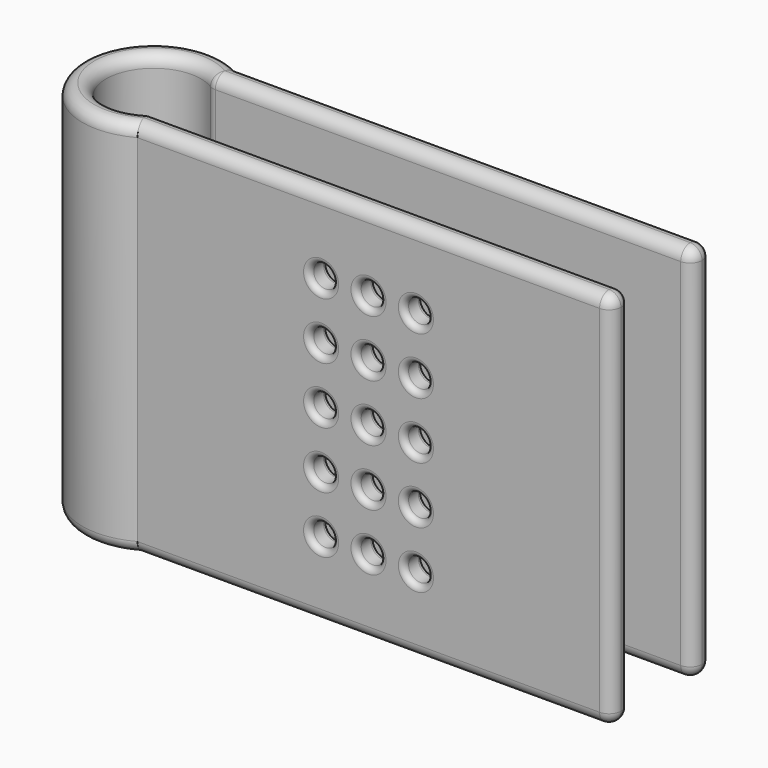
from build123d import *

# Parameters (mm, degrees)
F1_DEPTH = 25.4
F2_R     = 0.79374
F3_R     = 0.79375
F4_DEPTH = 8.9518078406
F5_R     = 0.381


# Not quite as in the source:
# - a fillet or chamfer is up to 0.001 mm smaller than in the source, because OpenCascade refuses the exact size


with BuildPart() as f1:
    # F0 (on Top) → F1 (new body)
    with BuildSketch(Plane.XY):
        with BuildLine():
            ThreePointArc((1.8211051854, -2.6008077406), (-3.175, 0), (1.8211051854, 2.6008077406))
            Line((1.8211051854, 2.6008077406), (2.7316577781, 3.9012116109))
            ThreePointArc((2.7316577781, 3.9012116109), (2.5034693369, 4.0514253701), (2.2670431226, 4.1883077406))
            ThreePointArc((2.2670431226, 4.1883077406), (-4.7625, 0), (2.2670431226, -4.1883077406))
            ThreePointArc((2.2670431226, -4.1883077406), (2.5034693369, -4.0514253701), (2.7316577781, -3.9012116109))
            Line((2.7316577781, -3.9012116109), (1.8211051854, -2.6008077406))
        make_face()
        with BuildLine():
            ThreePointArc((2.2670431226, 4.1883077406), (2.5034693369, 4.0514253701), (2.7316577781, 3.9012116109))
            ThreePointArc((2.7316577781, 3.9012116109), (3.4229686317, 3.3112976303), (3.989637245, 2.6008077406))
            Line((3.989637245, 2.6008077406), (34.0170431226, 2.6008077406))
            Line((34.0170431226, 2.6008077406), (34.0170431226, 4.1883077406))
            Line((34.0170431226, 4.1883077406), (2.2670431226, 4.1883077406))
        make_face()
        with BuildLine():
            Line((3.989637245, -2.6008077406), (1.8211051854, -2.6008077406))
            Line((1.8211051854, -2.6008077406), (2.7316577781, -3.9012116109))
            ThreePointArc((2.7316577781, -3.9012116109), (3.4229686317, -3.3112976303), (3.989637245, -2.6008077406))
        make_face()
        with BuildLine():
            ThreePointArc((3.989637245, -2.6008077406), (3.4229686317, -3.3112976303), (2.7316577781, -3.9012116109))
            ThreePointArc((2.7316577781, -3.9012116109), (2.5034693369, -4.0514253701), (2.2670431226, -4.1883077406))
            Line((2.2670431226, -4.1883077406), (34.0170431226, -4.1883077406))
            Line((34.0170431226, -4.1883077406), (34.0170431226, -2.6008077406))
            Line((34.0170431226, -2.6008077406), (3.989637245, -2.6008077406))
        make_face()
        with BuildLine():
            Line((2.7316577781, 3.9012116109), (1.8211051854, 2.6008077406))
            Line((1.8211051854, 2.6008077406), (3.989637245, 2.6008077406))
            ThreePointArc((3.989637245, 2.6008077406), (3.4229686317, 3.3112976303), (2.7316577781, 3.9012116109))
        make_face()
    extrude(amount=F1_DEPTH)

    # F2 (radius 0.79375 in the source; OpenCascade refuses exactly that, so slightly less here)
    f2_edges = [f1.edges().sort_by_distance(p)[0] for p in [
        (-3.175, 0, 25.4),
        (17.919074, 2.600808, 25.4),
        (34.017043, 3.394558, 25.4),
        (18.142043, 4.188308, 25.4),
        (-4.7625, 0, 25.4),
        (18.142043, -4.188308, 25.4),
        (34.017043, -3.394558, 25.4),
        (17.919074, -2.600808, 25.4),
        (-3.175, 0, 0),
        (17.919074, 2.600808, 0),
        (34.017043, 3.394558, 0),
        (18.142043, 4.188308, 0),
        (-4.7625, 0, 0),
        (18.142043, -4.188308, 0),
        (34.017043, -3.394558, 0),
        (17.919074, -2.600808, 0),
        (34.017043, 2.600808, 12.7),
        (34.017043, 4.188308, 12.7),
        (34.017043, -4.188308, 12.7),
        (34.017043, -2.600808, 12.7),
        (1.821105, -2.600808, 12.7),
        (1.821105, 2.600808, 12.7),
    ]]
    fillet(f2_edges, radius=F2_R)

    # F3 (on face) → F4 (cut, through all)
    with BuildSketch(Plane.XZ.offset(4.1883077406)):
        with Locations((17.7451681226, 12.7)):
            Circle(F3_R)
        with Locations((20.9201681226, 12.7000016774)):
            Circle(F3_R)
        with Locations((14.5701681226, 8.8900020029)):
            Circle(F3_R)
        with Locations((17.7451681226, 8.89)):
            Circle(F3_R)
        with Locations((20.9201681226, 8.8900016774)):
            Circle(F3_R)
        with Locations((17.7451681226, 5.08)):
            Circle(F3_R)
        with Locations((20.9201681226, 5.0800016774)):
            Circle(F3_R)
        with Locations((14.5701681226, 12.7000016774)):
            Circle(F3_R)
        with Locations((17.7451681226, 16.5100008387)):
            Circle(F3_R)
        with Locations((20.9201681226, 16.5100016774)):
            Circle(F3_R)
        with Locations((14.5701681226, 20.3200016774)):
            Circle(F3_R)
        with Locations((17.7451681226, 20.3200016774)):
            Circle(F3_R)
        with Locations((20.9201681226, 20.3200016774)):
            Circle(F3_R)
        with Locations((14.5701681226, 16.5100016774)):
            Circle(F3_R)
        with Locations((14.5701681226, 5.0800023283)):
            Circle(F3_R)
    extrude(amount=-F4_DEPTH, mode=Mode.SUBTRACT)

    # F5
    f5_edges = [f1.edges().sort_by_distance(p)[0] for p in [
        (13.776418, -4.188308, 5.080002),
        (15.363918, -3.394558, 5.080002),
        (13.776418, -2.600808, 5.080002),
        (13.776418, 2.600808, 5.080002),
        (15.363918, 3.394558, 5.080002),
        (13.776418, 4.188308, 5.080002),
        (16.951418, -4.188308, 5.08),
        (18.538918, -3.394558, 5.08),
        (16.951418, -2.600808, 5.08),
        (16.951418, 2.600808, 5.08),
        (18.538918, 3.394558, 5.08),
        (16.951418, 4.188308, 5.08),
        (20.126418, -4.188308, 5.080002),
        (21.713918, -3.394558, 5.080002),
        (20.126418, -2.600808, 5.080002),
        (20.126418, 2.600808, 5.080002),
        (21.713918, 3.394558, 5.080002),
        (20.126418, 4.188308, 5.080002),
        (20.126418, -4.188308, 8.890002),
        (21.713918, -3.394558, 8.890002),
        (20.126418, -2.600808, 8.890002),
        (20.126418, 2.600808, 8.890002),
        (21.713918, 3.394558, 8.890002),
        (20.126418, 4.188308, 8.890002),
        (16.951418, -4.188308, 8.89),
        (18.538918, -3.394558, 8.89),
        (16.951418, -2.600808, 8.89),
        (16.951418, 2.600808, 8.89),
        (18.538918, 3.394558, 8.89),
        (16.951418, 4.188308, 8.89),
        (13.776418, -4.188308, 8.890002),
        (15.363918, -3.394558, 8.890002),
        (13.776418, -2.600808, 8.890002),
        (13.776418, 2.600808, 8.890002),
        (15.363918, 3.394558, 8.890002),
        (13.776418, 4.188308, 8.890002),
        (13.776418, -4.188308, 12.700002),
        (15.363918, -3.394558, 12.700002),
        (13.776418, -2.600808, 12.700002),
        (13.776418, 2.600808, 12.700002),
        (15.363918, 3.394558, 12.700002),
        (13.776418, 4.188308, 12.700002),
        (16.951418, -4.188308, 12.7),
        (18.538918, -3.394558, 12.7),
        (16.951418, -2.600808, 12.7),
        (16.951418, 2.600808, 12.7),
        (18.538918, 3.394558, 12.7),
        (16.951418, 4.188308, 12.7),
        (20.126418, -4.188308, 12.700002),
        (21.713918, -3.394558, 12.700002),
        (20.126418, -2.600808, 12.700002),
        (20.126418, 2.600808, 12.700002),
        (21.713918, 3.394558, 12.700002),
        (20.126418, 4.188308, 12.700002),
        (20.126418, -4.188308, 16.510002),
        (21.713918, -3.394558, 16.510002),
        (20.126418, -2.600808, 16.510002),
        (20.126418, 2.600808, 16.510002),
        (21.713918, 3.394558, 16.510002),
        (20.126418, 4.188308, 16.510002),
        (16.951418, -4.188308, 16.510001),
        (18.538918, -3.394558, 16.510001),
        (16.951418, -2.600808, 16.510001),
        (16.951418, 2.600808, 16.510001),
        (18.538918, 3.394558, 16.510001),
        (16.951418, 4.188308, 16.510001),
        (13.776418, -4.188308, 16.510002),
        (15.363918, -3.394558, 16.510002),
        (13.776418, -2.600808, 16.510002),
        (13.776418, 2.600808, 16.510002),
        (15.363918, 3.394558, 16.510002),
        (13.776418, 4.188308, 16.510002),
        (20.126418, -4.188308, 20.320002),
        (21.713918, -3.394558, 20.320002),
        (20.126418, -2.600808, 20.320002),
        (20.126418, 2.600808, 20.320002),
        (21.713918, 3.394558, 20.320002),
        (20.126418, 4.188308, 20.320002),
        (16.951418, -4.188308, 20.320002),
        (18.538918, -3.394558, 20.320002),
        (16.951418, -2.600808, 20.320002),
        (16.951418, 2.600808, 20.320002),
        (18.538918, 3.394558, 20.320002),
        (16.951418, 4.188308, 20.320002),
        (13.776418, -4.188308, 20.320002),
        (15.363918, -3.394558, 20.320002),
        (13.776418, -2.600808, 20.320002),
        (13.776418, 2.600808, 20.320002),
        (15.363918, 3.394558, 20.320002),
        (13.776418, 4.188308, 20.320002),
    ]]
    fillet(f5_edges, radius=F5_R)


solid = f1.part
